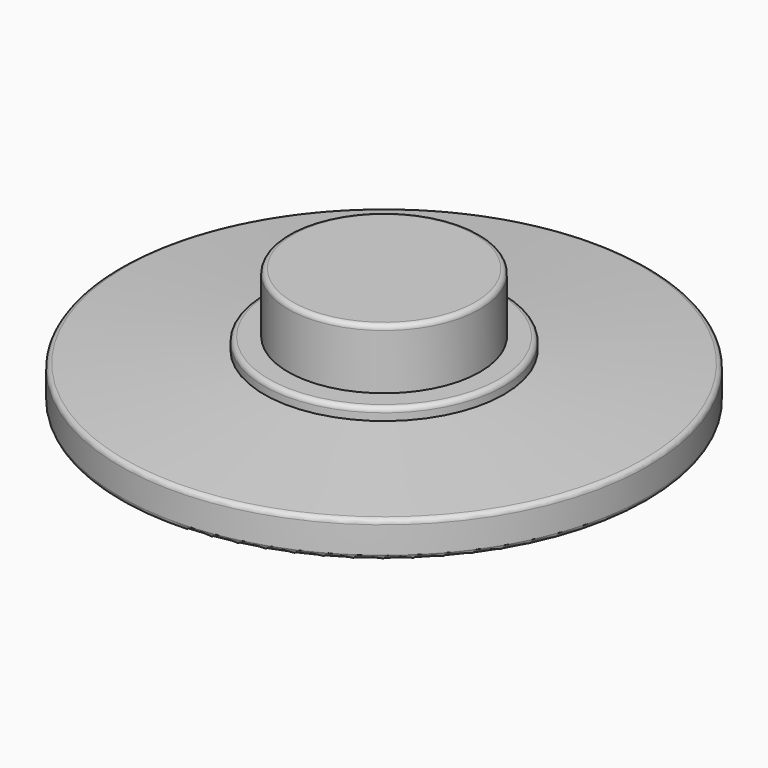
from build123d import *

# Parameters (mm, degrees)
F0_R     = 11
F1_DEPTH = 2
F2_R     = 5
F3_DEPTH = 0.5
F4_R     = 4
F5_DEPTH = 2.5
F6_SIZE2 = 0.49999
F6_SIZE  = 5.99999
F7_R     = 0.2


# Not quite as in the source:
# - a fillet or chamfer is up to 0.001 mm smaller than in the source, because OpenCascade refuses the exact size


with BuildPart() as f1:
    # F0 (on Top) → F1 (new body)
    with BuildSketch(Plane.XY):
        Circle(F0_R)
    extrude(amount=F1_DEPTH)

    # F2 (on face) → F3 (join)
    with BuildSketch(Plane.XY.offset(2)):
        Circle(F2_R)
    extrude(amount=F3_DEPTH)

    # F4 (on face) → F5 (join)
    with BuildSketch(Plane.XY.offset(2.5)):
        Circle(F4_R)
    extrude(amount=F5_DEPTH)

    # F6 (size 6 and 0.5 in the source; OpenCascade refuses exactly that, so slightly less here)
    f6_edges = [f1.edges().sort_by_distance(p)[0] for p in [
        (-11, 0, 2),
    ]]
    f6_side = f1.faces().sort_by_distance((-10.688873, 0, 2))[0]
    chamfer(f6_edges, length=F6_SIZE, length2=F6_SIZE2, reference=f6_side)

    # F7
    f7_edges = [f1.edges().sort_by_distance(p)[0] for p in [
        (-4, 0, 5),
        (-5, 0, 2.5),
        (-11, 0, 0),
        (-11, 0, 1.50001),
    ]]
    fillet(f7_edges, radius=F7_R)


solid = f1.part
